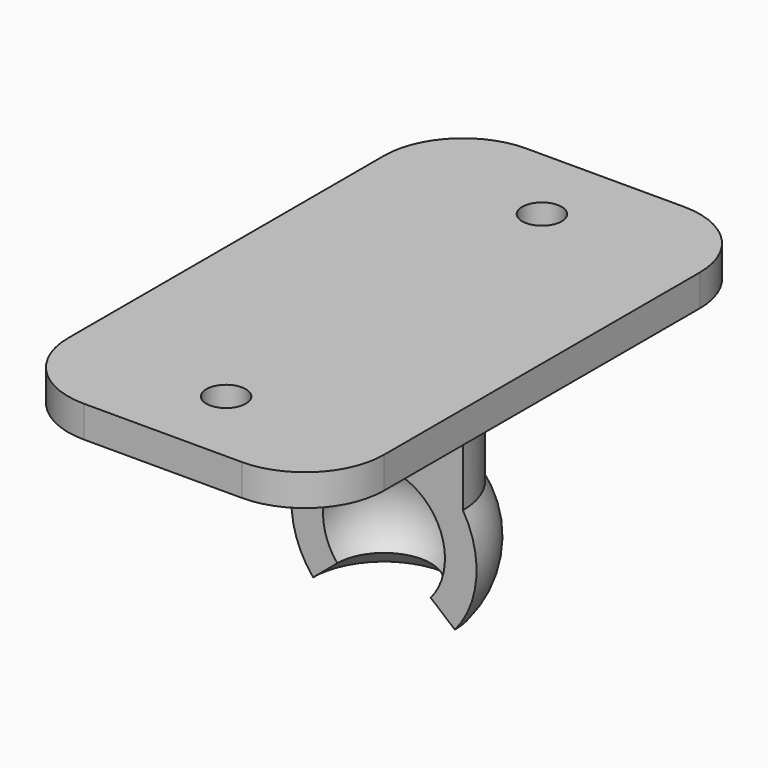
from build123d import *

# Parameters (mm, degrees)
F1_ANGLE = 180
F3_R     = 1.905
F4_DEPTH = 7.621
F5_W     = 25.4
F5_H     = 44.45
F6_DEPTH = 2.54
F7_R     = 6.35
F8_R     = 1.5875
F9_DEPTH = 21.1169539488


with BuildPart() as f1:
    # F0 (on Front) → F1 (revolve)
    with BuildSketch(Plane.XZ):
        with BuildLine():
            ThreePointArc((0, 4.9022), (4.4429020336, 2.0717592427), (3.7553030691, -3.1510734202))
            Line((3.7553030691, -3.1510734202), (5.7010559546, -4.7837539488))
            ThreePointArc((5.7010559546, -4.7837539488), (7.4214159865, -0.5558107544), (6.35, 3.8812164124))
            Line((6.35, 3.8812164124), (6.35, 7.3025))
            Line((6.35, 7.3025), (6.35, 12.5222))
            Line((6.35, 12.5222), (7.62, 13.7922))
            Line((7.62, 13.7922), (6.35, 13.7922))
            Line((6.35, 13.7922), (0, 13.7922))
            Line((0, 13.7922), (0, 7.4422))
            Line((0, 7.4422), (0, 4.9022))
        make_face()
    revolve(axis=Axis((0, 0, 10.6172), (0, 0, 1)), revolution_arc=F1_ANGLE)

    # F3 (on face) → F4 (cut, through all)
    with BuildSketch(Plane.XZ):
        with Locations((0, 9.9822)):
            Circle(F3_R)
    extrude(amount=-F4_DEPTH, mode=Mode.SUBTRACT)


with BuildPart() as f6:
    # F5 (on face) → F6 (new body)
    with BuildSketch(Plane.XY.offset(13.7922)):
        Rectangle(F5_W, F5_H)
        with BuildLine():
            ThreePointArc((-7.62, 0), (0, 7.62), (7.62, 0))
            Line((7.62, 0), (-7.62, 0))
        make_face(mode=Mode.SUBTRACT)
        with BuildLine():
            Line((-7.62, 0), (7.62, 0))
            ThreePointArc((7.62, 0), (0, 7.62), (-7.62, 0))
        make_face()
    extrude(amount=F6_DEPTH)

    # F7
    f7_edges = [f6.edges().sort_by_distance(p)[0] for p in [
        (12.7, 22.225, 15.0622),
        (-12.7, 22.225, 15.0622),
        (-12.7, -22.225, 15.0622),
        (12.7, -22.225, 15.0622),
    ]]
    fillet(f7_edges, radius=F7_R)

    # F8 (on face) → F9 (cut, through all)
    with BuildSketch(Plane.XY.offset(16.3322)):
        with Locations((0, 15.875)):
            Circle(F8_R)
        with Locations((0, -15.875)):
            Circle(F8_R)
    extrude(amount=-F9_DEPTH, mode=Mode.SUBTRACT)


solid = Compound([f1.part, f6.part])
